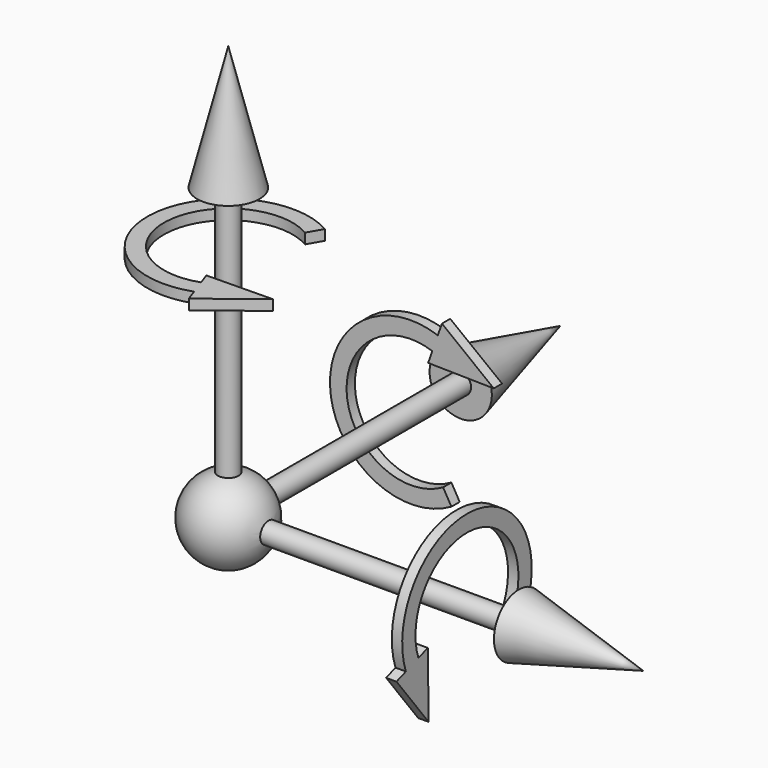
from build123d import *

# Parameters (mm, degrees)
F0_W              = 700
F0_H              = 25
F10_DEPTH         = 25
F10_COPIES_COUNT  = 2
F10_COPIES_ANGLE  = 270
F10_COPIES1_COUNT = 2
F10_COPIES1_ANGLE = 90


# Not quite as in the source:
# - a feature of the source that left no trace in its solid (it failed there, or was rolled back) is left out
# - a pattern or mirror of a feature is missing from the dataset's text; its kind, count and spacing are read off the source's solid


with BuildPart() as f1:
    # F0 (on Front) → F1 (revolve)
    with BuildSketch(Plane.XZ):
        Polygon((700, 25), (700, 0), (1000, 0), (700, 75), align=None)
        with Locations((350, 12.5)):
            Rectangle(F0_W, F0_H)
    revolve(axis=Axis((350, 0, 0), (-1, 0, 0)))

    # F2 (on Right) → F3 (revolve)
    with BuildSketch(Plane.YZ):
        Polygon((0, 0), (1000, 0), (700, 75), (700, 25), (0, 25), align=None)
    revolve(axis=Axis((0, 500, 0), (0, -1, 0)))

    # F4 (on Front) → F5 (revolve)
    with BuildSketch(Plane.XZ):
        Polygon((-25, 0), (0, 0), (0, 1000), (-75, 700), (-25, 700), align=None)
    revolve(axis=Axis((0, 0, 500), (0, 0, 1)))

    # F6 (on Right) → F7 (revolve)
    with BuildSketch(Plane.YZ):
        with BuildLine():
            Line((0, 100), (0, -100))
            ThreePointArc((0, -100), (100, 0), (0, 100))
        make_face()
    revolve(axis=Axis((0, 0, 0), (0, 0, -1)))


with BuildPart() as f10:
    # F9 (on offset) → F10 (new body)
    with BuildSketch(Plane.XY.offset(550)):
        with BuildLine():
            Line((77.5, 134.2339375866), (97.5, 168.874953738))
            ThreePointArc((97.5, 168.874953738), (-194.1661126327, 18.0144582243), (64.7672646877, -183.9298818161))
            Line((64.7672646877, -183.9298818161), (51.4816719313, -146.2006752897))
            ThreePointArc((51.4816719313, -146.2006752897), (-154.3371664516, 14.3191847424), (77.5, 134.2339375866))
        make_face()
        Polygon((51.4816719313, -146.2006752897), (64.7672646877, -183.9298818161), (74.7314592551, -212.2267867108), (199.6089927834, -115.2443057162), (41.5174773639, -117.9037703949), align=None)
    extrude(amount=F10_DEPTH)


with BuildPart() as f10_copies_1:
    # F10_copies: instance of F10
    add(f10.part.rotate(Axis((0, 0, 0), (1, 0, 0)), 1 * F10_COPIES_ANGLE / (F10_COPIES_COUNT - 1)))


with BuildPart() as f10_copies1_1:
    # F10_copies1: instance of F10
    add(f10.part.rotate(Axis((0, 0, 0), (0, 1, 0)), 1 * F10_COPIES1_ANGLE / (F10_COPIES1_COUNT - 1)))


solid = Compound([f1.part, f10.part, f10_copies_1.part, f10_copies1_1.part])
